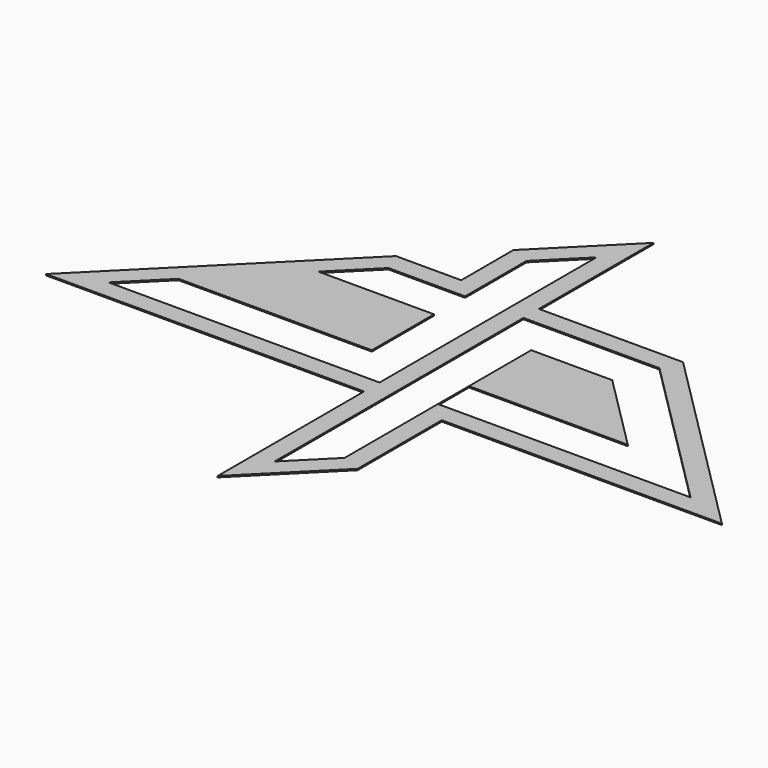
from build123d import *

# Parameters (mm, degrees)
F0_W     = 0.001
F0_H     = 60
F1_DEPTH = 2


# Not quite as in the source:
# - a feature names something its author has since deleted; it is built from what else it names


with BuildPart() as f1:
    # F0 (on Top) → F1 (new body)
    with BuildSketch(Plane.XY):
        Polygon((-409.5329046249, 667.7558401073), (-409.5329046249, 703.2591700554), (-409.5329046249, 710.1822469785), (-439.5329046249, 680.1822469785), (-439.5329046249, 637.7558401073), align=None)
        Polygon((-409.5329046249, 489.3550023332), (-409.5329046249, 667.7558401073), (-439.5329046249, 637.7558401073), (-439.5329046249, 219.3550023332), (-439.5329046249, 189.3550023332), (-439.5329046249, -93.071404538), (-409.5329046249, -63.071404538), (-409.5329046249, -20.6449976668), (-409.5329046249, 189.3550023332), (-409.5329046249, 279.3550023332), (-409.5329046249, 399.3550023332), (-409.5329046249, 459.3550023332), align=None)
        Polygon((-187.1064977537, 489.3550023332), (-409.5329046249, 489.3550023332), (-409.5329046249, 459.3550023332), (-199.5329046249, 459.3550023332), (-157.1064977537, 459.3550023332), align=None)
        Polygon((-499.5329046249, 577.7558401073), (-439.5329046249, 637.7558401073), (-439.5329046249, 680.1822469785), (-499.5329046249, 620.1822469785), (-499.5329046249, 579.3550023332), align=None)
        Polygon((-439.5329046249, 189.3550023332), (-439.5329046249, 219.3550023332), (-857.933742399, 219.3550023332), (-887.933742399, 189.3550023332), align=None)
        Polygon((-529.5329046249, 547.7558401073), (-499.5329046249, 577.7558401073), (-499.5329046249, 579.3550023332), (-499.5329046249, 620.1822469785), (-529.5329046249, 590.1822469785), align=None)
        Polygon((-499.5329046249, 459.3550023332), (-499.5329046249, 577.7558401073), (-529.5329046249, 547.7558401073), (-529.5329046249, 489.3550023332), (-587.933742399, 489.3550023332), (-617.933742399, 459.3550023332), align=None)
        Polygon((-157.1064977537, 459.3550023332), (-199.5329046249, 459.3550023332), (-139.5329046249, 399.3550023332), (40.4670953751, 219.3550023332), (-44.3857183673, 219.3550023332), (-349.5319046249, 219.3550023332), (-349.5329046249, 219.3550023332), (-349.5329046249, 189.3550023332), (-319.5329046249, 189.3550023332), (112.8935022463, 189.3550023332), align=None)
        Polygon((-887.933742399, 189.3550023332), (-857.933742399, 219.3550023332), (-900.3601492702, 219.3550023332), (-930.3601492702, 189.3550023332), align=None)
        Polygon((-900.3601492702, 219.3550023332), (-857.933742399, 219.3550023332), (-797.933742399, 279.3550023332), (-840.3601492702, 279.3550023332), align=None)
        Polygon((-224.3857183673, 399.3550023332), (-349.5329046249, 399.3550023332), (-349.5329046249, 279.3550023332), (-349.5319046249, 279.3550023332), (-104.3857183673, 279.3550023332), align=None)
        Polygon((-677.933742399, 399.3550023332), (-797.933742399, 279.3550023332), (-499.5329046249, 279.3550023332), (-499.5329046249, 399.3550023332), align=None)
        Polygon((-840.3601492702, 279.3550023332), (-797.933742399, 279.3550023332), (-677.933742399, 399.3550023332), (-720.3601492702, 399.3550023332), align=None)
        Polygon((-677.933742399, 399.3550023332), (-617.933742399, 459.3550023332), (-660.3601492702, 459.3550023332), (-720.3601492702, 399.3550023332), align=None)
        Polygon((-660.3601492702, 459.3550023332), (-617.933742399, 459.3550023332), (-587.933742399, 489.3550023332), (-630.3601492702, 489.3550023332), align=None)
        with Locations((-349.5324046249, 249.3550023332)):
            Rectangle(F0_W, F0_H)
        Polygon((-319.5329046249, 26.928595462), (-319.5329046249, 189.3550023332), (-349.5329046249, 189.3550023332), (-349.5329046249, 39.3550023332), (-349.5329046249, -3.071404538), align=None)
        Polygon((-409.5329046249, -20.6449976668), (-409.5329046249, -63.071404538), (-349.5329046249, -3.071404538), (-349.5329046249, 39.3550023332), align=None)
    extrude(amount=F1_DEPTH)


solid = f1.part
